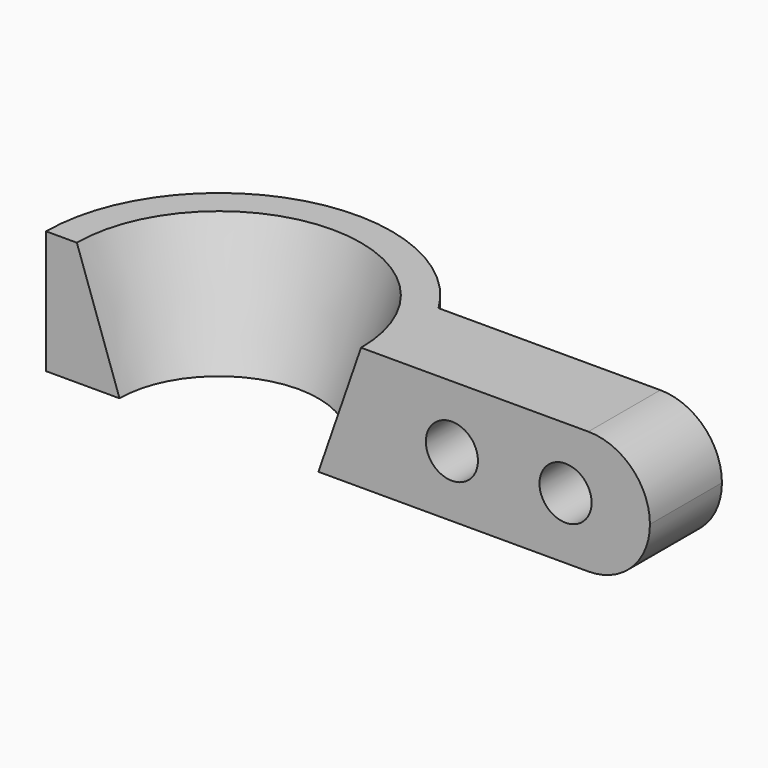
from build123d import *

# Parameters (mm, degrees)
F1_DEPTH = 52
F5_DEPTH = 25
F6_R     = 26
F7_R     = 25.99999


# Not quite as in the source:
# - a fillet or chamfer is up to 0.001 mm smaller than in the source, because OpenCascade refuses the exact size


with BuildPart() as f1:
    # F0 (on Top) → F1 (new body)
    with BuildSketch(Plane.XY):
        with BuildLine():
            Line((182, 38), (62.329768169, 38))
            ThreePointArc((62.329768169, 38), (-19.7348286497, 70.2818364741), (-73, 0))
            Line((-73, 0), (0, 0))
            Line((0, 0), (182, 0))
            Line((182, 0), (182, 38))
        make_face()
    extrude(amount=F1_DEPTH)

    # F2 (on face) → F3 (revolve, cut)
    with BuildSketch(Plane.XZ):
        Polygon((0, 52), (-60, 52), (-42, 0), (0, 0), align=None)
    revolve(axis=Axis((0, 0, 26), (0, 0, 1)), mode=Mode.SUBTRACT)

    # F4 (on face) → F5 (cut)
    with BuildSketch(Plane.XZ):
        with BuildLine():
            Line((87.3696654439, 26), (109.3696654439, 26))
            ThreePointArc((109.3696654439, 26), (98.3696654439, 37), (87.3696654439, 26))
        make_face()
        with BuildLine():
            ThreePointArc((157.3696654439, 26), (146.3696654439, 37), (135.3696654439, 26))
            Line((135.3696654439, 26), (157.3696654439, 26))
        make_face()
        with BuildLine():
            Line((157.3696654439, 26), (135.3696654439, 26))
            ThreePointArc((135.3696654439, 26), (146.3696654439, 15), (157.3696654439, 26))
        make_face()
        with BuildLine():
            ThreePointArc((87.3696654439, 26), (98.3696654439, 15), (109.3696654439, 26))
            Line((109.3696654439, 26), (87.3696654439, 26))
        make_face()
    extrude(amount=-F5_DEPTH, mode=Mode.SUBTRACT)

    # F6
    f6_edges = [f1.edges().sort_by_distance(p)[0] for p in [
        (182, 19, 52),
    ]]
    fillet(f6_edges, radius=F6_R)

    # F7 (radius 26 in the source; OpenCascade refuses exactly that, so slightly less here)
    f7_edges = [f1.edges().sort_by_distance(p)[0] for p in [
        (182, 19, 0),
    ]]
    fillet(f7_edges, radius=F7_R)


solid = f1.part
